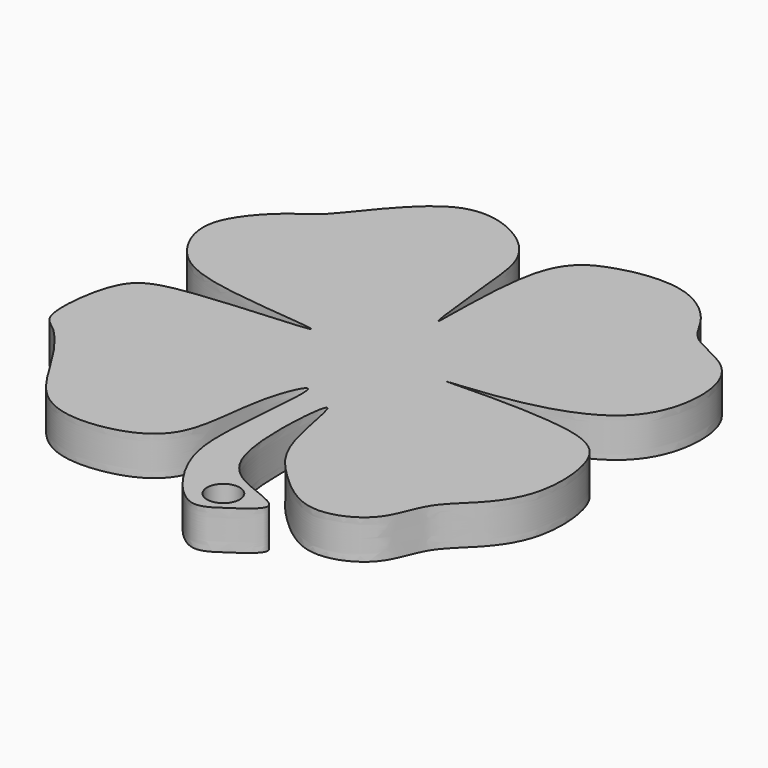
from build123d import *

# Parameters (mm, degrees)
F0_R     = 1.5
F1_DEPTH = 3.6


with BuildPart() as f1:
    # F0 (on Top) → F1 (new body)
    with BuildSketch(Plane.XY):
        with BuildLine():
            add(Edge.make_bspline(
                [(-30.6804964347, 31.582962714), (-29.1675241006, 33.1683116406), (-24.5766114637, 40.2041119836), (-17.7552043061, 37.7133351399), (-15.2448956288, 34.5130337453), (-14.9305064705, 30.6904965563), (-13.6106887962, 18.5451541561), (-14.3442713456, 35.0075738872), (-9.9487450503, 38.1266544345), (-3.2284013313, 39.0893520479), (0.8277993183, 35.7283365925), (1.8241774897, 32.7061701943), (6.4312643442, 31.4155236701), (8.459499043, 27.2718175176), (7.0729270519, 19.9046528379), (-1.2871097748, 17.0291239958), (-12.1454874012, 16.3606527779), (5.0115348488, 17.1588392772), (8.4087215997, 13.5116679061), (8.6705541856, 7.0469306097), (5.9973328421, 3.3029003142), (2.9728708099, 0.8856881591), (2.1857503326, -3.3699017834), (-3.1476545462, -5.7943429048), (-7.7562974509, -1.8824981318), (-10.780047028, 1.5581469324), (-11.9301777081, 11.8265548251), (-12.8524209858, -0.1105781927), (-10.5288130699, -4.7488661744), (-4.0243207571, -6.0981107197), (-7.7706271168, -8.5844472427), (-10.4860550532, -10.6001707727), (-15.0642090598, -4.6221073091), (-15.3576129259, 0.995038079), (-14.0183540343, 11.9838293904), (-16.7159094737, 6.0175211527), (-16.7347455052, -0.6842198121), (-19.7124095527, -3.8486596836), (-24.9619707202, -4.8734961624), (-29.195553996, -3.3631179401), (-31.8827564992, 1.7865724359), (-34.7545908947, 5.5928553158), (-36.8652956954, 6.4664289254), (-36.1149591658, 14.0722286464), (-32.5718884037, 16.2885824506), (-13.8708121692, 16.8343345652), (-30.7950542725, 17.6407765926), (-35.187087623, 20.2926504832), (-37.325976991, 25.6074724242), (-32.7268294715, 30.2927643508), (-31.4816804035, 30.7434522243), (-30.6804964347, 31.582962714)],
                knots=[0, 0, 0, 0, 0.026999185, 0.0484077675, 0.065039546, 0.0840025414, 0.1061960418, 0.1340810298, 0.1546259655, 0.1764535485, 0.1956059066, 0.2106087082, 0.2286424413, 0.2466072793, 0.2687031986, 0.2955772501, 0.3156255266, 0.3454275498, 0.3650849951, 0.3861544498, 0.4046908315, 0.4214988201, 0.4390111469, 0.4581913272, 0.478394237, 0.4988317716, 0.5196841966, 0.5432776965, 0.5645829712, 0.5828917435, 0.5976059263, 0.6124913414, 0.6338121384, 0.6570487017, 0.6811030666, 0.6968088938, 0.7203805666, 0.7376581895, 0.7572571934, 0.7750880091, 0.7961574612, 0.8149774419, 0.8270573228, 0.8491056078, 0.8684182172, 0.8977488788, 0.924559829, 0.9460336257, 0.9649165764, 0.9857027695, 1, 1, 1, 1], degree=3))
        make_face()
        with Locations((-9.3222688884, -6.987889763)):
            Circle(F0_R, mode=Mode.SUBTRACT)
    extrude(amount=F1_DEPTH)


solid = f1.part
